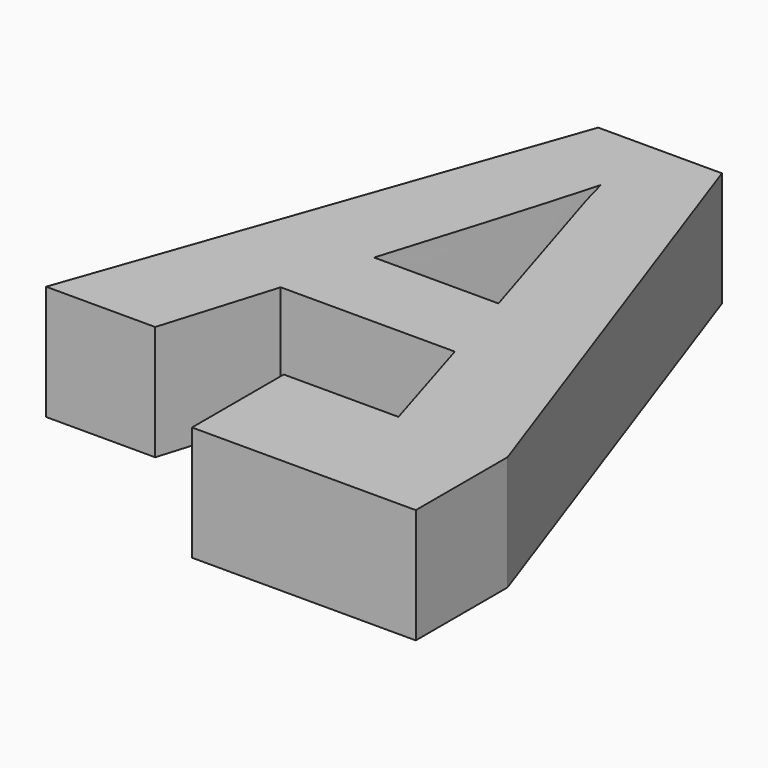
from build123d import *

# Parameters (mm, degrees)
F0_TEXT_SIZE = 148.1007474164
F1_DEPTH     = 25.4
F2_DEPTH     = 25.4
F3_DEPTH     = 25.4


# Not quite as in the source:
# - Text() gives the source's letters only with a copy of the font that has no kerning and outlines rounded to 1/6400 em; it was checked with that copy


with BuildPart() as f1:
    # F0 (on Top) → F1 (new body)
    with BuildSketch(Plane.XY):
        with Locations((-141.1163248122, -58.8642805815)):
            Text('A', F0_TEXT_SIZE, font='Open Sans', font_style=FontStyle.BOLD, text_align=(TextAlign.LEFT, TextAlign.BOTTOM))
    extrude(amount=F1_DEPTH)

    # F2 (add): a face of the model
    f2_faces = [f1.faces().sort_by_distance(p)[0] for p in [
        (-51.006276306, -58.8642805815, 12.7),
    ]]
    extrude(f2_faces, amount=F2_DEPTH)

    # F3 (add): a face of the model
    f3_faces = [f1.faces().sort_by_distance(p)[0] for p in [
        (-63.0857435171, -71.5642805815, 12.7),
    ]]
    extrude(f3_faces, amount=F3_DEPTH)


solid = f1.part
